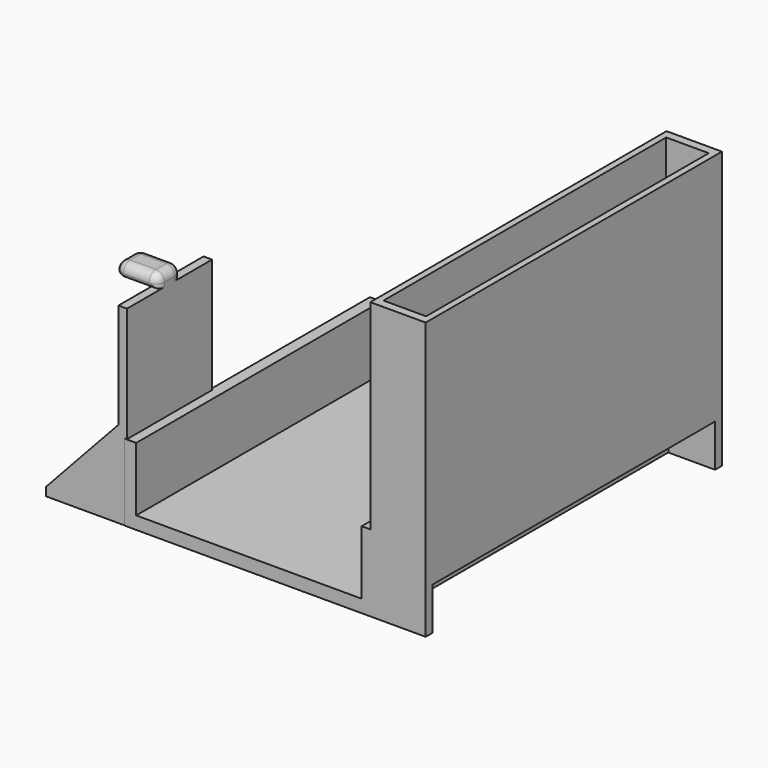
from build123d import *

# Parameters (mm, degrees)
F0_W      = 17
F0_H      = 25
F1_DEPTH  = 2
F0_W_2    = 2
F2_DEPTH  = 45
F3_W      = 2
F3_H      = 7
F4_DEPTH  = 3
F5_R      = 2
F6_R      = 2
F7_R      = 2
F8_R      = 2
F9_R      = 0.99999
F12_DEPTH = 2
F13_DEPTH = 2
F14_W     = 53
F14_H     = 68
F15_DEPTH = 3
F14_W_2   = 57
F14_H_2   = 72
F16_DEPTH = 23
F17_W     = 52.9679324031
F17_H     = 2
F18_DEPTH = 20
F19_DEPTH = 0.7
F21_DEPTH = 5
F22_W     = 87
F22_H     = 65
F23_DEPTH = 13
F25_W     = 83
F25_H     = 10
F26_DEPTH = 11
F24_W     = 10
F24_H     = 83
F27_DEPTH = 45
F28_DEPTH = 45
F29_DEPTH = 45


# Not quite as in the source:
# - a fillet or chamfer is up to 0.001 mm smaller than in the source, because OpenCascade refuses the exact size


with BuildPart() as f1:
    # F0 (on Top) → F1 (new body)
    with BuildSketch(Plane.XY):
        with Locations((22.646613881, -23.1278307736)):
            Rectangle(F0_W, F0_H)
    extrude(amount=F1_DEPTH)

    # F0 (on Top) → F2 (join)
    with BuildSketch(Plane.XY):
        with Locations((32.146613881, -23.1278307736)):
            Rectangle(F0_W_2, F0_H)
    extrude(amount=F2_DEPTH)

    # F3 (on face) → F4 (join)
    with BuildSketch(Plane.XY.offset(45)):
        Polygon((29.146613881, -26.6278307736), (31.146613881, -26.6278307736), (31.146613881, -19.6278307736), (23.146613881, -19.6278307736), (23.146613881, -25.5845747888), (23.146613881, -26.6278307736), align=None)
        with Locations((32.146613881, -23.1278307736)):
            Rectangle(F3_W, F3_H)
    extrude(amount=F4_DEPTH)

    # F5
    f5_edges = [f1.edges().sort_by_distance(p)[0] for p in [
        (23.146614, -23.127831, 48),
    ]]
    fillet(f5_edges, radius=F5_R)

    # F6
    f6_edges = [f1.edges().sort_by_distance(p)[0] for p in [
        (29.146614, -26.627831, 48),
    ]]
    fillet(f6_edges, radius=F6_R)

    # F7
    f7_edges = [f1.edges().sort_by_distance(p)[0] for p in [
        (29.146614, -19.627831, 48),
    ]]
    fillet(f7_edges, radius=F7_R)

    # F8
    f8_edges = [f1.edges().sort_by_distance(p)[0] for p in [
        (33.146614, -23.127831, 48),
    ]]
    fillet(f8_edges, radius=F8_R)

    # F9 (radius 1 in the source; OpenCascade refuses exactly that, so slightly less here)
    f9_edges = [f1.edges().sort_by_distance(p)[0] for p in [
        (23.146614, -23.127831, 45),
    ]]
    fillet(f9_edges, radius=F9_R)

    # F11 (on face) → F12 (join)
    with BuildSketch(Plane.XZ.offset(35.6278307736)):
        Polygon((31.146613881, 2), (31.146613881, 20.3421052632), (14.146613881, 2), align=None)
    extrude(amount=-F12_DEPTH)

    # F10 (on face) → F13 (join)
    with BuildSketch(Plane(origin=(0, -10.6278307736, 0), x_dir=(-1, 0, 0), z_dir=(0, 1, 0))):
        Polygon((-14.146613881, 2), (-31.146613881, 20.3421052632), (-31.146613881, 2), align=None)
    extrude(amount=-F13_DEPTH)


with BuildPart() as f15:
    # F14 (on Top) → F15 (new body)
    with BuildSketch(Plane.XY):
        with Locations((61.8922058344, 0.291702956)):
            Rectangle(F14_W, F14_H)
    extrude(amount=F15_DEPTH)

    # F14 (on Top) → F16 (join)
    with BuildSketch(Plane.XY):
        with Locations((61.8922058344, 0.291702956)):
            Rectangle(F14_W_2, F14_H_2)
        with Locations((61.8922058344, 0.291702956)):
            Rectangle(F14_W, F14_H, mode=Mode.SUBTRACT)
    extrude(amount=F16_DEPTH)

    # F17 (on face) → F18 (cut)
    with BuildSketch(Plane.XY.offset(23)):
        with Locations((61.8761720359, -34.708297044)):
            Rectangle(F17_W, F17_H)
    extrude(amount=-F18_DEPTH, mode=Mode.SUBTRACT)


with BuildPart() as f19:
    # F19 (new): a face of the model
    f19_faces = [f15.part.faces().sort_by_distance(p)[0] for p in [
        (33.3922058344, 0.291702956, 11.5),
    ]]
    extrude(f19_faces, amount=F19_DEPTH)


with BuildPart() as f1_1:
    add(f1.part)

    # F20: union F19, F15
    add(f19.part)
    add(f15.part)

    # F21 (cut): a face of the model
    f21_faces = [f1_1.faces().sort_by_distance(p)[0] for p in [
        (61.5422058344, 35.3690280403, 23),
    ]]
    extrude(f21_faces, amount=-F21_DEPTH, mode=Mode.SUBTRACT)

    # F22 (on face) → F23 (join)
    with BuildSketch(Plane.YZ.offset(90.3922058344)):
        with Locations((7.791702956, 32.5)):
            Rectangle(F22_W, F22_H)
    extrude(amount=F23_DEPTH)

    # F25 (on face) → F26 (cut)
    with BuildSketch(Plane.YZ.offset(103.3922058344)):
        with Locations((7.791702956, 5)):
            Rectangle(F25_W, F25_H)
    extrude(amount=-F26_DEPTH, mode=Mode.SUBTRACT)

    # F24 (on face) → F27 (join)
    with BuildSketch(Plane.XY.offset(65)):
        with Locations((96.8922058344, 7.791702956)):
            Rectangle(F24_W, F24_H)
    extrude(amount=-F27_DEPTH)

    # F24 (on face) → F28 (join)
    with BuildSketch(Plane.XY.offset(65)):
        with Locations((96.8922058344, 7.791702956)):
            Rectangle(F24_W, F24_H)
    extrude(amount=-F28_DEPTH)

    # F24 (on face) → F29 (cut)
    with BuildSketch(Plane.XY.offset(65)):
        with Locations((96.8922058344, 7.791702956)):
            Rectangle(F24_W, F24_H)
    extrude(amount=-F29_DEPTH, mode=Mode.SUBTRACT)


solid = f1_1.part
